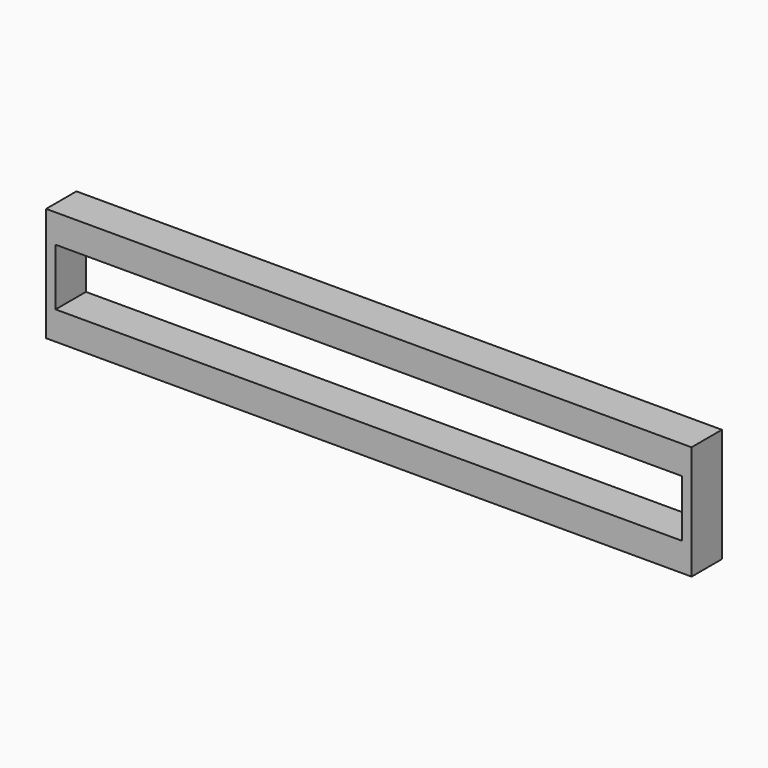
from build123d import *

# Parameters (mm, degrees)
F0_W     = 419.1
F0_H     = 38.1
F1_DEPTH = 12.7
F2_DEPTH = 25.4


# Not quite as in the source:
# - a feature names something its author has since deleted; it is built from what else it names


with BuildPart() as f1:
    # F0 (on Front) → F1 (new body)
    with BuildSketch(Plane.XZ):
        Polygon((215.9, 38.1), (-215.9, 38.1), (-215.9, 30.5130428595), (-215.9, -32.9869571405), (-215.9, -38.1), (215.9, -38.1), (215.9, -32.9869571405), (215.9, 30.5130428595), align=None)
        Rectangle(F0_W, F0_H, mode=Mode.SUBTRACT)
    extrude(amount=F1_DEPTH)

    # F0 (on Front) → F2 (join)
    with BuildSketch(Plane.XZ):
        Polygon((215.9, 38.1), (-215.9, 38.1), (-215.9, 30.5130428595), (-215.9, -32.9869571405), (-215.9, -38.1), (215.9, -38.1), (215.9, -32.9869571405), (215.9, 30.5130428595), align=None)
        Rectangle(F0_W, F0_H, mode=Mode.SUBTRACT)
    extrude(amount=F2_DEPTH)


solid = f1.part
